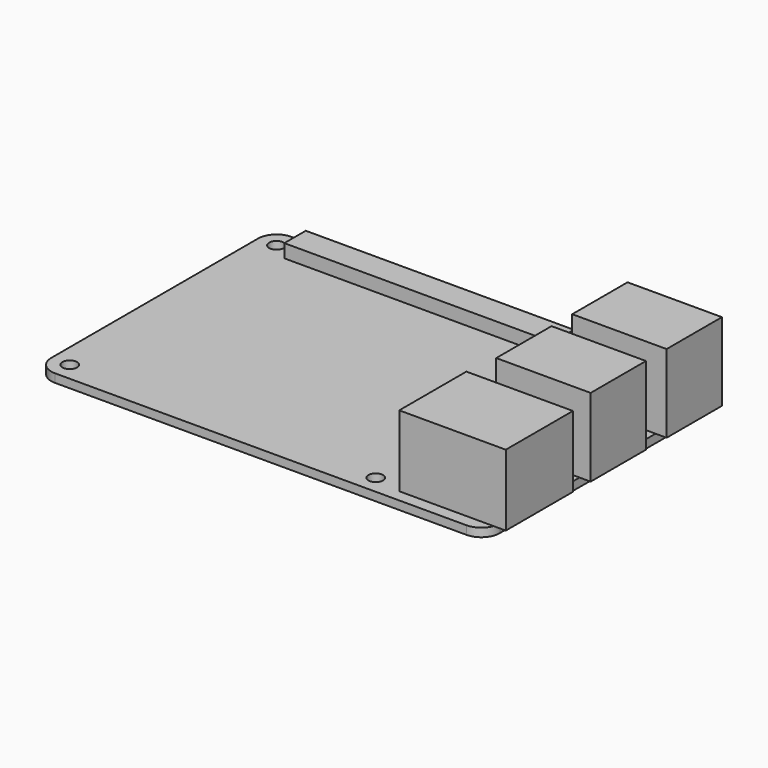
from build123d import *

# Parameters (mm, degrees)
F0_W        = 85
F0_H        = 56
F1_DEPTH    = 1.6
F2_D        = 2.8
F3_W        = 50.8
F3_H        = 5.08
F4_DEPTH    = 2.54
F5_W        = 17.8862189412
F5_H        = 13.1
F6_DEPTH    = 14.8
F7_W        = 20.1875766277
F7_H        = 15.9
F8_DEPTH    = 13.5
F9_T1_DEPTH = 19.1
F9_T3_DEPTH = 10.35


# Not quite as in the source:
# - a fillet or chamfer that OpenCascade refuses, or shapes differently, is made with other operations: its cross-section is extruded or revolved along the edge and cut away or added


with BuildPart() as f1:
    # F0 (on Top) → F1 (new body)
    with BuildSketch(Plane.XY):
        Rectangle(F0_W, F0_H)
    extrude(amount=F1_DEPTH)

    # F2 (through all)
    with Locations(Plane(origin=(0, 0, 0), x_dir=(1, 0, 0), z_dir=(0, 0, -1))):
        with Locations((-39, -24.5), (19, -24.5), (19, 24.5), (-39, 24.5)):
            Hole(F2_D / 2)

    # F3 (on face) → F4 (join)
    with BuildSketch(Plane.XY.offset(1.6)):
        with Locations((-10.1, 24.5)):
            Rectangle(F3_W, F3_H)
    extrude(amount=F4_DEPTH)

    # F5 (on face) → F6 (join)
    with BuildSketch(Plane.XY.offset(1.6)):
        with Locations((35.6568905294, 18.95)):
            Rectangle(F5_W, F5_H)
        with Locations((35.6568905294, 0.95)):
            Rectangle(F5_W, F5_H)
    extrude(amount=F6_DEPTH)

    # F7 (on face) → F8 (join)
    with BuildSketch(Plane.XY.offset(1.6)):
        with Locations((34.5062116861, -17.75)):
            Rectangle(F7_W, F7_H)
    extrude(amount=F8_DEPTH)

    # F9: fillet of radius 3.5 on 4 edges, made by hand

    # F9_s2 → F9_t1 (cut)
    with BuildSketch(Plane.XY.offset(-8.75)):
        with BuildLine():
            ThreePointArc((-39, -28), (-41.4748737342, -26.9748737342), (-42.5, -24.5))
            Line((-42.5, -24.5), (-42.5, -28))
            Line((-42.5, -28), (-39, -28))
        make_face()
        with BuildLine():
            ThreePointArc((-42.5, 24.5), (-41.4748737342, 26.9748737342), (-39, 28))
            Line((-39, 28), (-42.5, 28))
            Line((-42.5, 28), (-42.5, 24.5))
        make_face()
    extrude(amount=F9_T1_DEPTH, mode=Mode.SUBTRACT)

    # F9_s4 → F9_t3 (cut)
    with BuildSketch(Plane.XY.offset(-8.75)):
        with BuildLine():
            ThreePointArc((39, -28), (41.4748737342, -26.9748737342), (42.5, -24.5))
            Line((42.5, -24.5), (42.5, -28))
            Line((42.5, -28), (39, -28))
        make_face()
        with BuildLine():
            ThreePointArc((42.5, 24.5), (41.4748737342, 26.9748737342), (39, 28))
            Line((39, 28), (42.5, 28))
            Line((42.5, 28), (42.5, 24.5))
        make_face()
    extrude(amount=F9_T3_DEPTH, mode=Mode.SUBTRACT)


solid = f1.part
